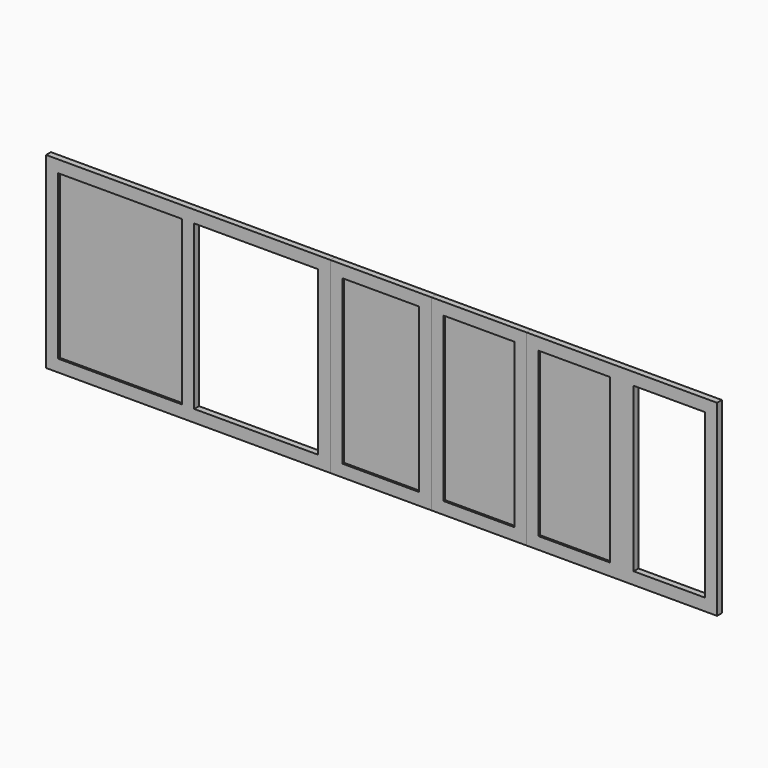
from build123d import *

# Parameters (mm, degrees)
F0_W     = 2810
F0_H     = 1855
F0_W_2   = 120
F0_H_2   = 1615
F1_DEPTH = 30
F0_W_3   = 1225
F2_DEPTH = 10
F0_W_4   = 1000
F0_W_5   = 760
F3_DEPTH = 30
F4_DEPTH = 10
F0_W_6   = 940
F0_W_7   = 700
F5_DEPTH = 30
F6_DEPTH = 10
F0_W_8   = 1885
F0_W_9   = 117.5
F7_DEPTH = 30
F0_W_10  = 705
F8_DEPTH = 10


with BuildPart() as f1:
    # F0 (on Front) → F1 (new body, symmetric)
    with BuildSketch(Plane.XZ):
        with Locations((1405, 927.5)):
            Rectangle(F0_W, F0_H)
        Polygon((120, 120), (120, 1735), (1345, 1735), (1465, 1735), (2690, 1735), (2690, 120), (1465, 120), (1345, 120), align=None, mode=Mode.SUBTRACT)
        with Locations((1405, 927.5)):
            Rectangle(F0_W_2, F0_H_2)
    extrude(amount=F1_DEPTH, both=True)


with BuildPart() as f2:
    # F0 (on Front) → F2 (new body, symmetric)
    with BuildSketch(Plane.XZ):
        with Locations((732.5, 927.5)):
            Rectangle(F0_W_3, F0_H_2)
    extrude(amount=F2_DEPTH, both=True)


with BuildPart() as f3:
    # F0 (on Front) → F3 (new body, symmetric)
    with BuildSketch(Plane.XZ):
        with Locations((3310, 927.5)):
            Rectangle(F0_W_4, F0_H)
        with Locations((3310, 927.5)):
            Rectangle(F0_W_5, F0_H_2, mode=Mode.SUBTRACT)
    extrude(amount=F3_DEPTH, both=True)


with BuildPart() as f4:
    # F0 (on Front) → F4 (new body, symmetric)
    with BuildSketch(Plane.XZ):
        with Locations((3310, 927.5)):
            Rectangle(F0_W_5, F0_H_2)
    extrude(amount=F4_DEPTH, both=True)


with BuildPart() as f5:
    # F0 (on Front) → F5 (new body, symmetric)
    with BuildSketch(Plane.XZ):
        with Locations((4280, 927.5)):
            Rectangle(F0_W_6, F0_H)
        with Locations((4280, 927.5)):
            Rectangle(F0_W_7, F0_H_2, mode=Mode.SUBTRACT)
    extrude(amount=F5_DEPTH, both=True)


with BuildPart() as f6:
    # F0 (on Front) → F6 (new body, symmetric)
    with BuildSketch(Plane.XZ):
        with Locations((4280, 927.5)):
            Rectangle(F0_W_7, F0_H_2)
    extrude(amount=F6_DEPTH, both=True)


with BuildPart() as f7:
    # F0 (on Front) → F7 (new body, symmetric)
    with BuildSketch(Plane.XZ):
        with Locations((5692.5, 927.5)):
            Rectangle(F0_W_8, F0_H)
        Polygon((5810, 1735), (6515, 1735), (6515, 120), (5810, 120), (5692.5, 120), (5575, 120), (4870, 120), (4870, 1735), (5575, 1735), (5692.5, 1735), align=None, mode=Mode.SUBTRACT)
        with Locations((5633.75, 927.5)):
            Rectangle(F0_W_9, F0_H_2)
        with Locations((5751.25, 927.5)):
            Rectangle(F0_W_9, F0_H_2)
    extrude(amount=F7_DEPTH, both=True)


with BuildPart() as f8:
    # F0 (on Front) → F8 (new body, symmetric)
    with BuildSketch(Plane.XZ):
        with Locations((5222.5, 927.5)):
            Rectangle(F0_W_10, F0_H_2)
    extrude(amount=F8_DEPTH, both=True)


solid = Compound([f1.part, f2.part, f3.part, f4.part, f5.part, f6.part, f7.part, f8.part])
